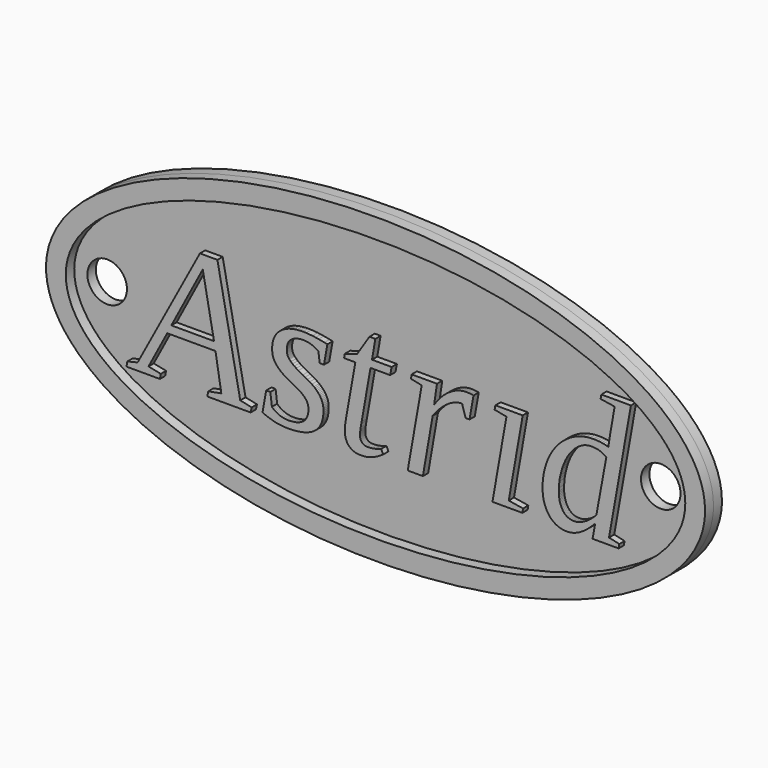
from build123d import *

# Parameters (mm, degrees)
F0_R     = 3
F1_DEPTH = 1.6
F2_DEPTH = 1.6
F3_DEPTH = 1


# Not quite as in the source:
# - a feature names something its author has since deleted; it is built from what else it names


with BuildPart() as f1:
    # F0 (on Front) → F1 (new body)
    with BuildSketch(Plane.XZ):
        with BuildLine():
            add(Edge.make_bspline(
                [(50, 0), (50, 39.8371685741), (-25, 19.918584287), (-100, 0), (-25, -19.918584287), (50, -39.8371685741), (50, 0)],
                knots=[0, 0, 0, 2.0943951024, 2.0943951024, 4.1887902048, 4.1887902048, 6.2831853072, 6.2831853072, 6.2831853072], degree=2, weights=[1, 0.5, 1, 0.5, 1, 0.5, 1]))
        make_face()
        with BuildLine():
            add(Edge.make_bspline(
                [(47, 0), (47, 34.6410161514), (-23.5, 17.3205080757), (-94, 0), (-23.5, -17.3205080757), (47, -34.6410161514), (47, 0)],
                knots=[0, 0, 0, 2.0943951024, 2.0943951024, 4.1887902048, 4.1887902048, 6.2831853072, 6.2831853072, 6.2831853072], degree=2, weights=[1, 0.5, 1, 0.5, 1, 0.5, 1]))
        make_face(mode=Mode.SUBTRACT)
        with BuildLine():
            add(Edge.make_bspline(
                [(47, 0), (47, 34.6410161514), (-23.5, 17.3205080757), (-94, 0), (-23.5, -17.3205080757), (47, -34.6410161514), (47, 0)],
                knots=[0, 0, 0, 2.0943951024, 2.0943951024, 4.1887902048, 4.1887902048, 6.2831853072, 6.2831853072, 6.2831853072], degree=2, weights=[1, 0.5, 1, 0.5, 1, 0.5, 1]))
        make_face()
        Polygon((-34.93235, -8.5991), (-33.05995, -8.9736), (-33.19865, -9.7087), (-38.27495, -9.7087), (-38.13625, -8.9736), (-36.58285, -8.5991), (-27.12375, 9.043), (-24.47465, 9.043), (-21.00725, -8.5991), (-19.27355, -8.9736), (-19.42615, -9.7087), (-26.01425, -9.7087), (-25.86165, -8.9736), (-23.87825, -8.5991), (-24.76595, -3.2316), (-32.08905, -3.2316), align=None, mode=Mode.SUBTRACT)
        Polygon((-8.39175, -5.6462), (-8.38525, -5.8807), (-8.39045, -6.1382), (-8.40605, -6.3874), (-8.43205, -6.628), (-8.46845, -6.8602), (-8.51525, -7.084), (-8.57245, -7.2993), (-8.64005, -7.5061), (-8.71805, -7.7045), (-8.80655, -7.8945), (-8.90535, -8.076), (-9.01455, -8.249), (-9.13415, -8.4136), (-9.26425, -8.5698), (-9.40465, -8.7175), (-9.55545, -8.8567), (-9.71665, -8.9875), (-9.88845, -9.1084), (-10.07105, -9.2215), (-10.26425, -9.3269), (-10.46825, -9.4244), (-10.68295, -9.5141), (-10.90845, -9.596), (-11.14455, -9.6701), (-11.39145, -9.7364), (-11.64905, -9.795), (-11.91745, -9.8457), (-12.19645, -9.8886), (-12.48625, -9.9237), (-13.09805, -9.9705), (-13.75275, -9.9861), (-14.36045, -9.9688), (-14.93515, -9.9167), (-15.47695, -9.8301), (-15.73545, -9.7737), (-15.98575, -9.7087), (-16.45825, -9.5631), (-16.67945, -9.4903), (-16.89075, -9.4174), (-17.09205, -9.3446), (-17.28345, -9.2718), (-17.46485, -9.199), (-17.63625, -9.1262), (-17.06755, -5.9916), (-16.44345, -5.9916), (-16.20765, -7.8918), (-16.11295, -7.9876), (-16.00915, -8.0808), (-15.89625, -8.1713), (-15.77425, -8.2593), (-15.64315, -8.3447), (-15.50295, -8.4275), (-15.35365, -8.5077), (-15.19515, -8.5853), (-15.02615, -8.6568), (-14.85195, -8.7188), (-14.67245, -8.7712), (-14.48785, -8.8141), (-14.29805, -8.8475), (-14.10295, -8.8713), (-13.90275, -8.8856), (-13.69725, -8.8904), (-13.38955, -8.8826), (-13.09045, -8.8592), (-12.80005, -8.8202), (-12.51835, -8.7656), (-12.38185, -8.732), (-12.24965, -8.6936), (-12.12175, -8.6505), (-11.99825, -8.6026), (-11.87905, -8.5499), (-11.76425, -8.4925), (-11.65365, -8.4303), (-11.54745, -8.3633), (-11.44625, -8.2877), (-11.35075, -8.2064), (-11.26075, -8.1195), (-11.17645, -8.027), (-11.09785, -7.9288), (-11.02475, -7.825), (-10.95735, -7.7156), (-10.89565, -7.6005), (-10.84035, -7.4757), (-10.79245, -7.3439), (-10.75195, -7.2052), (-10.71875, -7.0596), (-10.69295, -6.907), (-10.67455, -6.7475), (-10.66355, -6.5811), (-10.65985, -6.4077), (-10.66635, -6.2311), (-10.67445, -6.1456), (-10.68585, -6.0619), (-10.70045, -5.98), (-10.71835, -5.9), (-10.73945, -5.8218), (-10.76385, -5.7455), (-10.79145, -5.671), (-10.82235, -5.5983), (-10.85655, -5.5275), (-10.89385, -5.4585), (-10.93455, -5.3914), (-10.97845, -5.3261), (-11.02555, -5.2627), (-11.07595, -5.2011), (-11.17975, -5.0814), (-11.29005, -4.9653), (-11.40685, -4.8526), (-11.53015, -4.7434), (-11.65995, -4.6376), (-11.93905, -4.4365), (-12.08845, -4.3412), (-12.40045, -4.1496), (-13.06625, -3.782), (-13.41985, -3.6061), (-13.76745, -3.4266), (-14.10295, -3.2351), (-14.42635, -3.0313), (-14.73755, -2.8155), (-15.03045, -2.5762), (-15.29925, -2.3162), (-15.54365, -2.0353), (-15.76385, -1.7337), (-15.85815, -1.5726), (-15.93985, -1.4017), (-16.00895, -1.2207), (-16.06555, -1.0298), (-16.10955, -0.8289), (-16.14095, -0.618), (-16.15975, -0.3972), (-16.16605, -0.1664), (-16.16025, 0.0889), (-16.14265, 0.3346), (-16.11345, 0.5709), (-16.07245, 0.7975), (-16.01975, 1.0147), (-15.95545, 1.2223), (-15.87935, 1.4204), (-15.79155, 1.6089), (-15.69065, 1.7884), (-15.58185, 1.9591), (-15.46525, 2.1212), (-15.34085, 2.2747), (-15.20865, 2.4194), (-15.06865, 2.5555), (-14.92085, 2.6829), (-14.76525, 2.8017), (-14.59945, 2.9122), (-14.42805, 3.0149), (-14.25095, 3.1099), (-14.06825, 3.197), (-13.87995, 3.2763), (-13.68605, 3.3478), (-13.48645, 3.4115), (-13.28115, 3.4674), (-12.85295, 3.5585), (-12.41435, 3.6235), (-11.96535, 3.6625), (-11.50585, 3.6755), (-11.01095, 3.666), (-10.04695, 3.5897), (-9.57805, 3.5229), (-9.11775, 3.4501), (-8.22315, 3.2837), (-7.78885, 3.1901), (-8.30195, 0.2913), (-8.95385, 0.2913), (-9.14805, 1.7892), (-9.24855, 1.8737), (-9.35605, 1.9539), (-9.47055, 2.0298), (-9.59185, 2.1013), (-9.72015, 2.1685), (-9.85535, 2.2313), (-9.99755, 2.2898), (-10.14665, 2.344), (-10.29745, 2.396), (-10.45175, 2.4411), (-10.60955, 2.4792), (-10.77075, 2.5104), (-10.93545, 2.5347), (-11.10365, 2.552), (-11.27525, 2.5625), (-11.45045, 2.5659), (-11.72755, 2.5577), (-11.99045, 2.533), (-12.23905, 2.4918), (-12.35795, 2.465), (-12.47325, 2.4342), (-12.58505, 2.3992), (-12.69325, 2.36), (-12.79785, 2.3168), (-12.89895, 2.2695), (-12.99635, 2.218), (-13.09025, 2.1624), (-13.18055, 2.1027), (-13.26735, 2.0389), (-13.34965, 1.9725), (-13.42665, 1.9015), (-13.49825, 1.826), (-13.56465, 1.7459), (-13.62575, 1.6613), (-13.68145, 1.5721), (-13.73185, 1.4783), (-13.77705, 1.3801), (-13.81685, 1.2772), (-13.85135, 1.1699), (-13.88055, 1.0579), (-13.90445, 0.9414), (-13.92305, 0.8204), (-13.93635, 0.6948), (-13.94425, 0.5647), (-13.94695, 0.43), (-13.94065, 0.2636), (-13.93275, 0.1829), (-13.92175, 0.1041), (-13.90765, 0.0269), (-13.89035, -0.0485), (-13.86995, -0.1222), (-13.84635, -0.1941), (-13.81965, -0.2644), (-13.78985, -0.3328), (-13.75685, -0.3996), (-13.72065, -0.4646), (-13.68145, -0.5279), (-13.63895, -0.5894), (-13.59345, -0.6492), (-13.54475, -0.7073), (-13.32365, -0.9318), (-13.07665, -1.1477), (-12.80355, -1.3549), (-12.50445, -1.5534), (-12.18725, -1.7406), (-11.52145, -2.1151), (-11.17305, -2.3023), (-10.81845, -2.4896), (-10.47605, -2.6907), (-10.14575, -2.9056), (-9.82765, -3.1345), (-9.67505, -3.2554), (-9.52945, -3.3824), (-9.39075, -3.5155), (-9.25905, -3.6546), (-9.13415, -3.7998), (-9.01625, -3.9511), (-8.90535, -4.1084), (-8.80135, -4.2718), (-8.70375, -4.4395), (-8.61925, -4.6168), (-8.54775, -4.8036), (-8.48925, -5), (-8.44375, -5.2058), (-8.41125, -5.4213), align=None, mode=Mode.SUBTRACT)
        Polygon((-2.83555, -7.2163), (-2.83665, -7.2954), (-2.83545, -7.3722), (-2.83195, -7.4467), (-2.82595, -7.5187), (-2.81755, -7.5884), (-2.80685, -7.6557), (-2.79375, -7.7206), (-2.77825, -7.7831), (-2.76035, -7.8432), (-2.74015, -7.901), (-2.71745, -7.9564), (-2.69245, -8.0093), (-2.66505, -8.0599), (-2.63525, -8.1082), (-2.60305, -8.154), (-2.56845, -8.1975), (-2.53155, -8.2385), (-2.49105, -8.2755), (-2.44915, -8.31), (-2.40605, -8.3422), (-2.36165, -8.372), (-2.31595, -8.3994), (-2.26885, -8.4245), (-2.22055, -8.4471), (-2.17095, -8.4674), (-2.12005, -8.4852), (-2.06775, -8.5007), (-2.01425, -8.5139), (-1.95945, -8.5246), (-1.90325, -8.5329), (-1.84585, -8.5389), (-1.78715, -8.5425), (-1.72715, -8.5437), (-1.43495, -8.5367), (-1.15495, -8.5159), (-0.88715, -8.4812), (-0.63145, -8.4327), (-0.38085, -8.372), (0.12535, -8.2194), (0.38105, -8.1276), (0.67235, -8.7794), (0.30995, -9.0204), (-0.06965, -9.2441), (-0.46665, -9.4504), (-0.88105, -9.6394), (-1.09275, -9.7206), (-1.31185, -9.7911), (-1.53835, -9.8506), (-1.77215, -9.8994), (-2.01335, -9.9373), (-2.26195, -9.9644), (-2.51785, -9.9807), (-2.78115, -9.9861), (-2.92465, -9.9831), (-3.06375, -9.974), (-3.19855, -9.9588), (-3.32905, -9.9375), (-3.45515, -9.9102), (-3.57695, -9.8769), (-3.69445, -9.8374), (-3.80755, -9.7919), (-3.91635, -9.7445), (-4.02075, -9.6922), (-4.12095, -9.6352), (-4.21675, -9.5735), (-4.30815, -9.5069), (-4.39525, -9.4356), (-4.47805, -9.3596), (-4.55655, -9.2787), (-4.62715, -9.1936), (-4.69345, -9.1045), (-4.75545, -9.0115), (-4.81305, -8.9147), (-4.86645, -8.8139), (-4.91535, -8.7092), (-4.96005, -8.6006), (-5.00035, -8.4882), (-5.06105, -8.2472), (-5.10435, -7.9958), (-5.13035, -7.734), (-5.13905, -7.4618), (-5.13465, -7.2538), (-5.12165, -7.0319), (-5.10005, -6.7961), (-5.06965, -6.5464), (-5.03415, -6.2924), (-4.95785, -5.8001), (-4.91715, -5.5617), (-3.54405, 2.1637), (-5.24995, 2.1637), (-5.13905, 2.7878), (-3.29435, 3.3287), (-1.39425, 6.283), (-0.50655, 6.283), (-1.01975, 3.3287), (1.96225, 3.3287), (1.74035, 2.1637), (-1.24165, 2.1637), (-2.58705, -5.4507), (-2.63985, -5.7299), (-2.73005, -6.2569), (-2.76735, -6.5048), (-2.78355, -6.6234), (-2.79765, -6.7363), (-2.80955, -6.8435), (-2.81935, -6.9452), (-2.82695, -7.0412), (-2.83235, -7.1315), align=None, mode=Mode.SUBTRACT)
        Polygon((13.14785, 3.6722), (13.29435, 3.6755), (13.43655, 3.6729), (13.58565, 3.6651), (13.74165, 3.6521), (13.90465, 3.6339), (13.98505, 3.6267), (14.05985, 3.6191), (14.12895, 3.6111), (14.16145, 3.607), (14.19245, 3.6027), (14.22205, 3.5983), (14.25035, 3.5938), (14.27715, 3.5892), (14.30255, 3.5845), (14.32655, 3.5796), (14.34915, 3.5747), (14.37035, 3.5697), (14.39005, 3.5645), (13.77985, 0.1526), (13.18345, 0.1526), (12.65635, 1.914), (12.50385, 1.9101), (12.35125, 1.8984), (12.19865, 1.8789), (12.04615, 1.8516), (11.89355, 1.8165), (11.74095, 1.7736), (11.58845, 1.7229), (11.43585, 1.6644), (11.13335, 1.5283), (10.83605, 1.3697), (10.54385, 1.1885), (10.25695, 0.9848), (9.97525, 0.7681), (9.69865, 0.534), (9.42735, 0.2826), (9.16125, 0.0139), (8.90295, -0.2678), (8.41745, -0.8573), (8.19035, -1.165), (6.70635, -9.7087), (4.40395, -9.7087), (6.52605, 2.3579), (4.88945, 2.7046), (5.00035, 3.3287), (8.84225, 3.3287), (8.41225, 0.3884), (8.69315, 0.7915), (8.98095, 1.1686), (9.27565, 1.5196), (9.57735, 1.8447), (9.88945, 2.1429), (10.20145, 2.4134), (10.51355, 2.6561), (10.82565, 2.871), (11.13765, 3.0592), (11.44975, 3.2213), (11.76185, 3.3574), (12.07385, 3.4674), (12.38945, 3.5585), (12.69805, 3.6235), (12.84975, 3.6462), (12.99965, 3.6625), align=None, mode=Mode.SUBTRACT)
        Polygon((21.85265, 3.3287), (19.73055, -8.7378), (21.90815, -9.0846), (21.79715, -9.7087), (17.26185, -9.7087), (19.38385, 2.3579), (17.59465, 2.7046), (17.70565, 3.3287), align=None, mode=Mode.SUBTRACT)
        with Locations((-42, 0)):
            Circle(F0_R, mode=Mode.SUBTRACT)
        Polygon((22.71065, 7.6626), (22.71255, 7.5867), (22.71065, 7.5109), (22.70475, 7.4359), (22.69505, 7.3618), (22.68135, 7.2885), (22.66385, 7.2161), (22.64235, 7.1446), (22.61695, 7.074), (22.58775, 7.0042), (22.55845, 6.9392), (22.52615, 6.8759), (22.49085, 6.8144), (22.45255, 6.7545), (22.41115, 6.6965), (22.36665, 6.6401), (22.31925, 6.5855), (22.26875, 6.5326), (22.21565, 6.4819), (22.16035, 6.4338), (22.10295, 6.3883), (22.04335, 6.3454), (21.98155, 6.3051), (21.91765, 6.2674), (21.85155, 6.2323), (21.78325, 6.1998), (21.71355, 6.1738), (21.64285, 6.1512), (21.57135, 6.1321), (21.49895, 6.1165), (21.42575, 6.1044), (21.35165, 6.0957), (21.27665, 6.0905), (21.20075, 6.0888), (21.12495, 6.0905), (21.04995, 6.0957), (20.97585, 6.1044), (20.90255, 6.1165), (20.83015, 6.1321), (20.75865, 6.1512), (20.68805, 6.1738), (20.61825, 6.1998), (20.48995, 6.2674), (20.36855, 6.3454), (20.25415, 6.4338), (20.14665, 6.5326), (20.04785, 6.6401), (19.95945, 6.7545), (19.88145, 6.8759), (19.81385, 7.0042), (19.78785, 7.074), (19.76525, 7.1446), (19.74615, 7.2161), (19.73055, 7.2885), (19.71845, 7.3618), (19.70975, 7.4359), (19.70455, 7.5109), (19.70285, 7.5867), (19.70455, 7.6626), (19.70975, 7.7376), (19.71845, 7.8117), (19.73055, 7.8849), (19.74615, 7.9573), (19.76525, 8.0288), (19.78785, 8.0995), (19.81385, 8.1692), (19.84635, 8.2375), (19.88145, 8.3036), (19.91915, 8.3675), (19.95945, 8.4293), (20.00235, 8.4889), (20.04785, 8.5463), (20.09595, 8.6016), (20.14665, 8.6547), (20.19955, 8.7052), (20.25415, 8.7526), (20.31055, 8.7971), (20.36855, 8.8385), (20.42845, 8.8768), (20.48995, 8.9121), (20.55325, 8.9444), (20.61825, 8.9737), (20.68805, 9.0029), (20.75865, 9.0283), (20.83015, 9.0497), (20.90255, 9.0673), (20.97585, 9.081), (21.04995, 9.0907), (21.12495, 9.0966), (21.20075, 9.0985), (21.27665, 9.0966), (21.35165, 9.0907), (21.42575, 9.081), (21.49895, 9.0673), (21.57135, 9.0497), (21.64285, 9.0283), (21.71355, 9.0029), (21.78325, 8.9737), (21.85155, 8.9444), (21.91765, 8.9121), (21.98155, 8.8768), (22.04335, 8.8385), (22.10295, 8.7971), (22.16035, 8.7526), (22.21565, 8.7052), (22.26875, 8.6547), (22.31925, 8.6016), (22.36665, 8.5463), (22.41115, 8.4889), (22.45255, 8.4293), (22.49085, 8.3675), (22.52615, 8.3036), (22.55845, 8.2375), (22.58775, 8.1692), (22.61695, 8.0995), (22.64235, 8.0288), (22.66385, 7.9573), (22.68135, 7.8849), (22.69505, 7.8117), (22.70475, 7.7376), align=None, mode=Mode.SUBTRACT)
        Polygon((34.62115, 3.4146), (34.86305, 3.3426), (34.86485, 3.364), (34.86695, 3.3864), (34.86925, 3.4099), (34.87175, 3.4345), (34.87735, 3.4869), (34.88385, 3.5437), (34.89125, 3.6048), (34.89945, 3.6703), (34.90855, 3.7401), (34.91855, 3.8142), (34.94015, 3.9746), (34.98875, 4.3005), (35.01565, 4.4661), (35.04245, 4.6377), (35.09105, 4.9706), (35.11275, 5.1318), (35.12635, 5.2098), (35.13955, 5.2844), (35.15235, 5.3554), (35.16475, 5.4231), (35.17665, 5.4872), (35.18815, 5.5479), (35.19915, 5.6051), (35.20975, 5.6588), (35.80615, 9.043), (33.67025, 9.3759), (33.78125, 10), (38.27495, 10), (34.94625, -8.7378), (36.51355, -9.0846), (36.40255, -9.7087), (32.44975, -9.7087), (32.85195, -7.545), (32.56225, -7.8409), (32.27545, -8.118), (31.99185, -8.3766), (31.71115, -8.6165), (31.43355, -8.8377), (31.15895, -9.0404), (30.88745, -9.2243), (30.61895, -9.3897), (30.35325, -9.5327), (30.09015, -9.6567), (29.82965, -9.7616), (29.57175, -9.8474), (29.31645, -9.9141), (29.06385, -9.9618), (28.81375, -9.9904), (28.56625, -10), (28.36055, -9.995), (28.15965, -9.98), (27.96355, -9.9551), (27.77225, -9.9202), (27.58565, -9.8754), (27.40375, -9.8205), (27.22675, -9.7557), (27.05445, -9.681), (26.88755, -9.5969), (26.72675, -9.5041), (26.57205, -9.4027), (26.42335, -9.2926), (26.28075, -9.1739), (26.14425, -9.0464), (26.01375, -8.9103), (25.88945, -8.7656), (25.77125, -8.6089), (25.65965, -8.444), (25.55455, -8.2708), (25.45595, -8.0894), (25.36385, -7.8998), (25.27825, -7.7019), (25.19915, -7.4958), (25.12655, -7.2815), (25.06485, -7.0596), (25.01125, -6.8308), (24.96595, -6.595), (24.90015, -6.1026), (24.86715, -5.5825), (24.86305, -5.312), (24.87955, -4.72), (24.92895, -4.1366), (25.01125, -3.5619), (25.12655, -2.9958), (25.27225, -2.4358), (25.44555, -1.8932), (25.64665, -1.3679), (25.87555, -0.8599), (26.13035, -0.3718), (26.40955, 0.0937), (26.71295, 0.5366), (27.04055, 0.957), (27.39775, 1.3584), (27.77565, 1.7303), (28.17445, 2.0727), (28.59395, 2.3856), (29.03265, 2.6734), (29.48855, 2.9265), (29.96185, 3.145), (30.45255, 3.3287), (30.96485, 3.4744), (31.48925, 3.5784), (32.02585, 3.6408), (32.57455, 3.6616), (32.91265, 3.6564), (33.23335, 3.6408), (33.53675, 3.6148), (33.82285, 3.5784), (34.10105, 3.5325), (34.36725, 3.4778), align=None, mode=Mode.SUBTRACT)
        with Locations((42, 0)):
            Circle(F0_R, mode=Mode.SUBTRACT)
        Polygon((34.86485, 3.364), (34.86305, 3.3426), (34.62115, 3.4146), (34.36725, 3.4778), (34.10105, 3.5325), (33.82285, 3.5784), (33.53675, 3.6148), (33.23335, 3.6408), (32.91265, 3.6564), (32.57455, 3.6616), (32.02585, 3.6408), (31.48925, 3.5784), (30.96485, 3.4744), (30.45255, 3.3287), (29.96185, 3.145), (29.48855, 2.9265), (29.03265, 2.6734), (28.59395, 2.3856), (28.17445, 2.0727), (27.77565, 1.7303), (27.39775, 1.3584), (27.04055, 0.957), (26.71295, 0.5366), (26.40955, 0.0937), (26.13035, -0.3718), (25.87555, -0.8599), (25.64665, -1.3679), (25.44555, -1.8932), (25.27225, -2.4358), (25.12655, -2.9958), (25.01125, -3.5619), (24.92895, -4.1366), (24.87955, -4.72), (24.86305, -5.312), (24.86715, -5.5825), (24.90015, -6.1026), (24.96595, -6.595), (25.01125, -6.8308), (25.06485, -7.0596), (25.12655, -7.2815), (25.19915, -7.4958), (25.27825, -7.7019), (25.36385, -7.8998), (25.45595, -8.0894), (25.55455, -8.2708), (25.65965, -8.444), (25.77125, -8.6089), (25.88945, -8.7656), (26.01375, -8.9103), (26.14425, -9.0464), (26.28075, -9.1739), (26.42335, -9.2926), (26.57205, -9.4027), (26.72675, -9.5041), (26.88755, -9.5969), (27.05445, -9.681), (27.22675, -9.7557), (27.40375, -9.8205), (27.58565, -9.8754), (27.77225, -9.9202), (27.96355, -9.9551), (28.15965, -9.98), (28.36055, -9.995), (28.56625, -10), (28.81375, -9.9904), (29.06385, -9.9618), (29.31645, -9.9141), (29.57175, -9.8474), (29.82965, -9.7616), (30.09015, -9.6567), (30.35325, -9.5327), (30.61895, -9.3897), (30.88745, -9.2243), (31.15895, -9.0404), (31.43355, -8.8377), (31.71115, -8.6165), (31.99185, -8.3766), (32.27545, -8.118), (32.56225, -7.8409), (32.85195, -7.545), (32.44975, -9.7087), (36.40255, -9.7087), (36.51355, -9.0846), (34.94625, -8.7378), (38.27495, 10), (33.78125, 10), (33.67025, 9.3759), (35.80615, 9.043), (35.20975, 5.6588), (35.19915, 5.6051), (35.18815, 5.5479), (35.17665, 5.4872), (35.16475, 5.4231), (35.15235, 5.3554), (35.13955, 5.2844), (35.12635, 5.2098), (35.11275, 5.1318), (35.09105, 4.9706), (35.04245, 4.6377), (35.01565, 4.4661), (34.98875, 4.3005), (34.94015, 3.9746), (34.91855, 3.8142), (34.90855, 3.7401), (34.89945, 3.6703), (34.89125, 3.6048), (34.88385, 3.5437), (34.87735, 3.4869), (34.87175, 3.4345), (34.86925, 3.4099), (34.86695, 3.3864), align=None)
        Polygon((34.29955, 2.051), (34.54405, 1.9002), (33.03225, -6.3384), (32.81965, -6.5609), (32.38795, -6.9684), (32.16885, -7.1532), (31.94765, -7.3255), (31.72415, -7.4852), (31.49855, -7.6324), (31.27085, -7.767), (31.04735, -7.884), (30.82785, -7.9854), (30.61225, -8.0712), (30.40045, -8.1414), (30.19265, -8.196), (29.98875, -8.2351), (29.78875, -8.2585), (29.59255, -8.2663), (29.48535, -8.2634), (29.37845, -8.255), (29.27205, -8.2409), (29.16615, -8.2212), (29.06055, -8.1958), (28.95545, -8.1648), (28.85075, -8.1282), (28.74655, -8.086), (28.64725, -8.0376), (28.55065, -7.9828), (28.45655, -7.9215), (28.36515, -7.8536), (28.27625, -7.7793), (28.19005, -7.6985), (28.10635, -7.6111), (28.02535, -7.5173), (27.95075, -7.4135), (27.87965, -7.3032), (27.81205, -7.1864), (27.74795, -7.0631), (27.68725, -6.9333), (27.63005, -6.7969), (27.57625, -6.6541), (27.52605, -6.5048), (27.48055, -6.3449), (27.44105, -6.1771), (27.40765, -6.0016), (27.38035, -5.8183), (27.35915, -5.6271), (27.34395, -5.4282), (27.33485, -5.2214), (27.33185, -5.0069), (27.34135, -4.5622), (27.41765, -3.6676), (27.48445, -3.2177), (27.57625, -2.7704), (27.81205, -1.8966), (27.95595, -1.4701), (28.11635, -1.0541), (28.29235, -0.6518), (28.48385, -0.2635), (28.69105, 0.111), (28.91995, 0.4664), (29.16265, 0.7975), (29.41925, 1.1044), (29.68965, 1.387), (29.82985, 1.522), (30.11945, 1.7699), (30.42105, 1.9884), (30.73485, 2.1774), (30.89635, 2.2608), (31.06085, 2.3356), (31.22835, 2.4004), (31.39885, 2.4552), (31.57245, 2.5), (31.74915, 2.5349), (31.92875, 2.5599), (32.11145, 2.5748), (32.29715, 2.5798), (32.47745, 2.577), (32.65085, 2.5685), (32.81725, 2.5544), (32.97675, 2.5347), (33.12935, 2.5094), (33.27495, 2.4784), (33.41365, 2.4417), (33.54545, 2.3995), (33.80025, 2.3007), (34.05165, 2.1845), align=None, mode=Mode.SUBTRACT)
        Polygon((-33.19865, -9.7087), (-33.05995, -8.9736), (-34.93235, -8.5991), (-32.08905, -3.2316), (-24.76595, -3.2316), (-23.87825, -8.5991), (-25.86165, -8.9736), (-26.01425, -9.7087), (-19.42615, -9.7087), (-19.27355, -8.9736), (-21.00725, -8.5991), (-24.47465, 9.043), (-27.12375, 9.043), (-36.58285, -8.5991), (-38.13625, -8.9736), (-38.27495, -9.7087), align=None)
        Polygon((-31.46495, -1.9833), (-26.69385, 7.0458), (-24.98785, -1.9833), align=None, mode=Mode.SUBTRACT)
        Polygon((33.03225, -6.3384), (34.54405, 1.9002), (34.29955, 2.051), (34.05165, 2.1845), (33.80025, 2.3007), (33.54545, 2.3995), (33.41365, 2.4417), (33.27495, 2.4784), (33.12935, 2.5094), (32.97675, 2.5347), (32.81725, 2.5544), (32.65085, 2.5685), (32.47745, 2.577), (32.29715, 2.5798), (32.11145, 2.5748), (31.92875, 2.5599), (31.74915, 2.5349), (31.57245, 2.5), (31.39885, 2.4552), (31.22835, 2.4004), (31.06085, 2.3356), (30.89635, 2.2608), (30.73485, 2.1774), (30.42105, 1.9884), (30.11945, 1.7699), (29.82985, 1.522), (29.68965, 1.387), (29.41925, 1.1044), (29.16265, 0.7975), (28.91995, 0.4664), (28.69105, 0.111), (28.48385, -0.2635), (28.29235, -0.6518), (28.11635, -1.0541), (27.95595, -1.4701), (27.81205, -1.8966), (27.57625, -2.7704), (27.48445, -3.2177), (27.41765, -3.6676), (27.34135, -4.5622), (27.33185, -5.0069), (27.33485, -5.2214), (27.34395, -5.4282), (27.35915, -5.6271), (27.38035, -5.8183), (27.40765, -6.0016), (27.44105, -6.1771), (27.48055, -6.3449), (27.52605, -6.5048), (27.57625, -6.6541), (27.63005, -6.7969), (27.68725, -6.9333), (27.74795, -7.0631), (27.81205, -7.1864), (27.87965, -7.3032), (27.95075, -7.4135), (28.02535, -7.5173), (28.10635, -7.6111), (28.19005, -7.6985), (28.27625, -7.7793), (28.36515, -7.8536), (28.45655, -7.9215), (28.55065, -7.9828), (28.64725, -8.0376), (28.74655, -8.086), (28.85075, -8.1282), (28.95545, -8.1648), (29.06055, -8.1958), (29.16615, -8.2212), (29.27205, -8.2409), (29.37845, -8.255), (29.48535, -8.2634), (29.59255, -8.2663), (29.78875, -8.2585), (29.98875, -8.2351), (30.19265, -8.196), (30.40045, -8.1414), (30.61225, -8.0712), (30.82785, -7.9854), (31.04735, -7.884), (31.27085, -7.767), (31.49855, -7.6324), (31.72415, -7.4852), (31.94765, -7.3255), (32.16885, -7.1532), (32.38795, -6.9684), (32.81965, -6.5609), align=None)
        Polygon((-8.39045, -6.1382), (-8.38525, -5.8807), (-8.39175, -5.6462), (-8.41125, -5.4213), (-8.44375, -5.2058), (-8.48925, -5), (-8.54775, -4.8036), (-8.61925, -4.6168), (-8.70375, -4.4395), (-8.80135, -4.2718), (-8.90535, -4.1084), (-9.01625, -3.9511), (-9.13415, -3.7998), (-9.25905, -3.6546), (-9.39075, -3.5155), (-9.52945, -3.3824), (-9.67505, -3.2554), (-9.82765, -3.1345), (-10.14575, -2.9056), (-10.47605, -2.6907), (-10.81845, -2.4896), (-11.17305, -2.3023), (-11.52145, -2.1151), (-12.18725, -1.7406), (-12.50445, -1.5534), (-12.80355, -1.3549), (-13.07665, -1.1477), (-13.32365, -0.9318), (-13.54475, -0.7073), (-13.59345, -0.6492), (-13.63895, -0.5894), (-13.68145, -0.5279), (-13.72065, -0.4646), (-13.75685, -0.3996), (-13.78985, -0.3328), (-13.81965, -0.2644), (-13.84635, -0.1941), (-13.86995, -0.1222), (-13.89035, -0.0485), (-13.90765, 0.0269), (-13.92175, 0.1041), (-13.93275, 0.1829), (-13.94065, 0.2636), (-13.94695, 0.43), (-13.94425, 0.5647), (-13.93635, 0.6948), (-13.92305, 0.8204), (-13.90445, 0.9414), (-13.88055, 1.0579), (-13.85135, 1.1699), (-13.81685, 1.2772), (-13.77705, 1.3801), (-13.73185, 1.4783), (-13.68145, 1.5721), (-13.62575, 1.6613), (-13.56465, 1.7459), (-13.49825, 1.826), (-13.42665, 1.9015), (-13.34965, 1.9725), (-13.26735, 2.0389), (-13.18055, 2.1027), (-13.09025, 2.1624), (-12.99635, 2.218), (-12.89895, 2.2695), (-12.79785, 2.3168), (-12.69325, 2.36), (-12.58505, 2.3992), (-12.47325, 2.4342), (-12.35795, 2.465), (-12.23905, 2.4918), (-11.99045, 2.533), (-11.72755, 2.5577), (-11.45045, 2.5659), (-11.27525, 2.5625), (-11.10365, 2.552), (-10.93545, 2.5347), (-10.77075, 2.5104), (-10.60955, 2.4792), (-10.45175, 2.4411), (-10.29745, 2.396), (-10.14665, 2.344), (-9.99755, 2.2898), (-9.85535, 2.2313), (-9.72015, 2.1685), (-9.59185, 2.1013), (-9.47055, 2.0298), (-9.35605, 1.9539), (-9.24855, 1.8737), (-9.14805, 1.7892), (-8.95385, 0.2913), (-8.30195, 0.2913), (-7.78885, 3.1901), (-8.22315, 3.2837), (-9.11775, 3.4501), (-9.57805, 3.5229), (-10.04695, 3.5897), (-11.01095, 3.666), (-11.50585, 3.6755), (-11.96535, 3.6625), (-12.41435, 3.6235), (-12.85295, 3.5585), (-13.28115, 3.4674), (-13.48645, 3.4115), (-13.68605, 3.3478), (-13.87995, 3.2763), (-14.06825, 3.197), (-14.25095, 3.1099), (-14.42805, 3.0149), (-14.59945, 2.9122), (-14.76525, 2.8017), (-14.92085, 2.6829), (-15.06865, 2.5555), (-15.20865, 2.4194), (-15.34085, 2.2747), (-15.46525, 2.1212), (-15.58185, 1.9591), (-15.69065, 1.7884), (-15.79155, 1.6089), (-15.87935, 1.4204), (-15.95545, 1.2223), (-16.01975, 1.0147), (-16.07245, 0.7975), (-16.11345, 0.5709), (-16.14265, 0.3346), (-16.16025, 0.0889), (-16.16605, -0.1664), (-16.15975, -0.3972), (-16.14095, -0.618), (-16.10955, -0.8289), (-16.06555, -1.0298), (-16.00895, -1.2207), (-15.93985, -1.4017), (-15.85815, -1.5726), (-15.76385, -1.7337), (-15.54365, -2.0353), (-15.29925, -2.3162), (-15.03045, -2.5762), (-14.73755, -2.8155), (-14.42635, -3.0313), (-14.10295, -3.2351), (-13.76745, -3.4266), (-13.41985, -3.6061), (-13.06625, -3.782), (-12.40045, -4.1496), (-12.08845, -4.3412), (-11.93905, -4.4365), (-11.65995, -4.6376), (-11.53015, -4.7434), (-11.40685, -4.8526), (-11.29005, -4.9653), (-11.17975, -5.0814), (-11.07595, -5.2011), (-11.02555, -5.2627), (-10.97845, -5.3261), (-10.93455, -5.3914), (-10.89385, -5.4585), (-10.85655, -5.5275), (-10.82235, -5.5983), (-10.79145, -5.671), (-10.76385, -5.7455), (-10.73945, -5.8218), (-10.71835, -5.9), (-10.70045, -5.98), (-10.68585, -6.0619), (-10.67445, -6.1456), (-10.66635, -6.2311), (-10.65985, -6.4077), (-10.66355, -6.5811), (-10.67455, -6.7475), (-10.69295, -6.907), (-10.71875, -7.0596), (-10.75195, -7.2052), (-10.79245, -7.3439), (-10.84035, -7.4757), (-10.89565, -7.6005), (-10.95735, -7.7156), (-11.02475, -7.825), (-11.09785, -7.9288), (-11.17645, -8.027), (-11.26075, -8.1195), (-11.35075, -8.2064), (-11.44625, -8.2877), (-11.54745, -8.3633), (-11.65365, -8.4303), (-11.76425, -8.4925), (-11.87905, -8.5499), (-11.99825, -8.6026), (-12.12175, -8.6505), (-12.24965, -8.6936), (-12.38185, -8.732), (-12.51835, -8.7656), (-12.80005, -8.8202), (-13.09045, -8.8592), (-13.38955, -8.8826), (-13.69725, -8.8904), (-13.90275, -8.8856), (-14.10295, -8.8713), (-14.29805, -8.8475), (-14.48785, -8.8141), (-14.67245, -8.7712), (-14.85195, -8.7188), (-15.02615, -8.6568), (-15.19515, -8.5853), (-15.35365, -8.5077), (-15.50295, -8.4275), (-15.64315, -8.3447), (-15.77425, -8.2593), (-15.89625, -8.1713), (-16.00915, -8.0808), (-16.11295, -7.9876), (-16.20765, -7.8918), (-16.44345, -5.9916), (-17.06755, -5.9916), (-17.63625, -9.1262), (-17.46485, -9.199), (-17.28345, -9.2718), (-17.09205, -9.3446), (-16.89075, -9.4174), (-16.67945, -9.4903), (-16.45825, -9.5631), (-15.98575, -9.7087), (-15.73545, -9.7737), (-15.47695, -9.8301), (-14.93515, -9.9167), (-14.36045, -9.9688), (-13.75275, -9.9861), (-13.09805, -9.9705), (-12.48625, -9.9237), (-12.19645, -9.8886), (-11.91745, -9.8457), (-11.64905, -9.795), (-11.39145, -9.7364), (-11.14455, -9.6701), (-10.90845, -9.596), (-10.68295, -9.5141), (-10.46825, -9.4244), (-10.26425, -9.3269), (-10.07105, -9.2215), (-9.88845, -9.1084), (-9.71665, -8.9875), (-9.55545, -8.8567), (-9.40465, -8.7175), (-9.26425, -8.5698), (-9.13415, -8.4136), (-9.01455, -8.249), (-8.90535, -8.076), (-8.80655, -7.8945), (-8.71805, -7.7045), (-8.64005, -7.5061), (-8.57245, -7.2993), (-8.51525, -7.084), (-8.46845, -6.8602), (-8.43205, -6.628), (-8.40605, -6.3874), align=None)
        Polygon((-2.83545, -7.3722), (-2.83665, -7.2954), (-2.83555, -7.2163), (-2.83235, -7.1315), (-2.82695, -7.0412), (-2.81935, -6.9452), (-2.80955, -6.8435), (-2.79765, -6.7363), (-2.78355, -6.6234), (-2.76735, -6.5048), (-2.73005, -6.2569), (-2.63985, -5.7299), (-2.58705, -5.4507), (-1.24165, 2.1637), (1.74035, 2.1637), (1.96225, 3.3287), (-1.01975, 3.3287), (-0.50655, 6.283), (-1.39425, 6.283), (-3.29435, 3.3287), (-5.13905, 2.7878), (-5.24995, 2.1637), (-3.54405, 2.1637), (-4.91715, -5.5617), (-4.95785, -5.8001), (-5.03415, -6.2924), (-5.06965, -6.5464), (-5.10005, -6.7961), (-5.12165, -7.0319), (-5.13465, -7.2538), (-5.13905, -7.4618), (-5.13035, -7.734), (-5.10435, -7.9958), (-5.06105, -8.2472), (-5.00035, -8.4882), (-4.96005, -8.6006), (-4.91535, -8.7092), (-4.86645, -8.8139), (-4.81305, -8.9147), (-4.75545, -9.0115), (-4.69345, -9.1045), (-4.62715, -9.1936), (-4.55655, -9.2787), (-4.47805, -9.3596), (-4.39525, -9.4356), (-4.30815, -9.5069), (-4.21675, -9.5735), (-4.12095, -9.6352), (-4.02075, -9.6922), (-3.91635, -9.7445), (-3.80755, -9.7919), (-3.69445, -9.8374), (-3.57695, -9.8769), (-3.45515, -9.9102), (-3.32905, -9.9375), (-3.19855, -9.9588), (-3.06375, -9.974), (-2.92465, -9.9831), (-2.78115, -9.9861), (-2.51785, -9.9807), (-2.26195, -9.9644), (-2.01335, -9.9373), (-1.77215, -9.8994), (-1.53835, -9.8506), (-1.31185, -9.7911), (-1.09275, -9.7206), (-0.88105, -9.6394), (-0.46665, -9.4504), (-0.06965, -9.2441), (0.30995, -9.0204), (0.67235, -8.7794), (0.38105, -8.1276), (0.12535, -8.2194), (-0.38085, -8.372), (-0.63145, -8.4327), (-0.88715, -8.4812), (-1.15495, -8.5159), (-1.43495, -8.5367), (-1.72715, -8.5437), (-1.78715, -8.5425), (-1.84585, -8.5389), (-1.90325, -8.5329), (-1.95945, -8.5246), (-2.01425, -8.5139), (-2.06775, -8.5007), (-2.12005, -8.4852), (-2.17095, -8.4674), (-2.22055, -8.4471), (-2.26885, -8.4245), (-2.31595, -8.3994), (-2.36165, -8.372), (-2.40605, -8.3422), (-2.44915, -8.31), (-2.49105, -8.2755), (-2.53155, -8.2385), (-2.56845, -8.1975), (-2.60305, -8.154), (-2.63525, -8.1082), (-2.66505, -8.0599), (-2.69245, -8.0093), (-2.71745, -7.9564), (-2.74015, -7.901), (-2.76035, -7.8432), (-2.77825, -7.7831), (-2.79375, -7.7206), (-2.80685, -7.6557), (-2.81755, -7.5884), (-2.82595, -7.5187), (-2.83195, -7.4467), align=None)
        Polygon((13.43655, 3.6729), (13.29435, 3.6755), (13.14785, 3.6722), (12.99965, 3.6625), (12.84975, 3.6462), (12.69805, 3.6235), (12.38945, 3.5585), (12.07385, 3.4674), (11.76185, 3.3574), (11.44975, 3.2213), (11.13765, 3.0592), (10.82565, 2.871), (10.51355, 2.6561), (10.20145, 2.4134), (9.88945, 2.1429), (9.57735, 1.8447), (9.27565, 1.5196), (8.98095, 1.1686), (8.69315, 0.7915), (8.41225, 0.3884), (8.84225, 3.3287), (5.00035, 3.3287), (4.88945, 2.7046), (6.52605, 2.3579), (4.40395, -9.7087), (6.70635, -9.7087), (8.19035, -1.165), (8.41745, -0.8573), (8.90295, -0.2678), (9.16125, 0.0139), (9.42735, 0.2826), (9.69865, 0.534), (9.97525, 0.7681), (10.25695, 0.9848), (10.54385, 1.1885), (10.83605, 1.3697), (11.13335, 1.5283), (11.43585, 1.6644), (11.58845, 1.7229), (11.74095, 1.7736), (11.89355, 1.8165), (12.04615, 1.8516), (12.19865, 1.8789), (12.35125, 1.8984), (12.50385, 1.9101), (12.65635, 1.914), (13.18345, 0.1526), (13.77985, 0.1526), (14.39005, 3.5645), (14.37035, 3.5697), (14.34915, 3.5747), (14.32655, 3.5796), (14.30255, 3.5845), (14.27715, 3.5892), (14.25035, 3.5938), (14.22205, 3.5983), (14.19245, 3.6027), (14.16145, 3.607), (14.12895, 3.6111), (14.05985, 3.6191), (13.98505, 3.6267), (13.90465, 3.6339), (13.74165, 3.6521), (13.58565, 3.6651), align=None)
        Polygon((21.90815, -9.0846), (19.73055, -8.7378), (21.85265, 3.3287), (17.70565, 3.3287), (17.59465, 2.7046), (19.38385, 2.3579), (17.26185, -9.7087), (21.79715, -9.7087), align=None)
        Polygon((-24.98785, -1.9833), (-26.69385, 7.0458), (-31.46495, -1.9833), align=None)
        Polygon((22.71065, 7.5109), (22.71255, 7.5867), (22.71065, 7.6626), (22.70475, 7.7376), (22.69505, 7.8117), (22.68135, 7.8849), (22.66385, 7.9573), (22.64235, 8.0288), (22.61695, 8.0995), (22.58775, 8.1692), (22.55845, 8.2375), (22.52615, 8.3036), (22.49085, 8.3675), (22.45255, 8.4293), (22.41115, 8.4889), (22.36665, 8.5463), (22.31925, 8.6016), (22.26875, 8.6547), (22.21565, 8.7052), (22.16035, 8.7526), (22.10295, 8.7971), (22.04335, 8.8385), (21.98155, 8.8768), (21.91765, 8.9121), (21.85155, 8.9444), (21.78325, 8.9737), (21.71355, 9.0029), (21.64285, 9.0283), (21.57135, 9.0497), (21.49895, 9.0673), (21.42575, 9.081), (21.35165, 9.0907), (21.27665, 9.0966), (21.20075, 9.0985), (21.12495, 9.0966), (21.04995, 9.0907), (20.97585, 9.081), (20.90255, 9.0673), (20.83015, 9.0497), (20.75865, 9.0283), (20.68805, 9.0029), (20.61825, 8.9737), (20.55325, 8.9444), (20.48995, 8.9121), (20.42845, 8.8768), (20.36855, 8.8385), (20.31055, 8.7971), (20.25415, 8.7526), (20.19955, 8.7052), (20.14665, 8.6547), (20.09595, 8.6016), (20.04785, 8.5463), (20.00235, 8.4889), (19.95945, 8.4293), (19.91915, 8.3675), (19.88145, 8.3036), (19.84635, 8.2375), (19.81385, 8.1692), (19.78785, 8.0995), (19.76525, 8.0288), (19.74615, 7.9573), (19.73055, 7.8849), (19.71845, 7.8117), (19.70975, 7.7376), (19.70455, 7.6626), (19.70285, 7.5867), (19.70455, 7.5109), (19.70975, 7.4359), (19.71845, 7.3618), (19.73055, 7.2885), (19.74615, 7.2161), (19.76525, 7.1446), (19.78785, 7.074), (19.81385, 7.0042), (19.88145, 6.8759), (19.95945, 6.7545), (20.04785, 6.6401), (20.14665, 6.5326), (20.25415, 6.4338), (20.36855, 6.3454), (20.48995, 6.2674), (20.61825, 6.1998), (20.68805, 6.1738), (20.75865, 6.1512), (20.83015, 6.1321), (20.90255, 6.1165), (20.97585, 6.1044), (21.04995, 6.0957), (21.12495, 6.0905), (21.20075, 6.0888), (21.27665, 6.0905), (21.35165, 6.0957), (21.42575, 6.1044), (21.49895, 6.1165), (21.57135, 6.1321), (21.64285, 6.1512), (21.71355, 6.1738), (21.78325, 6.1998), (21.85155, 6.2323), (21.91765, 6.2674), (21.98155, 6.3051), (22.04335, 6.3454), (22.10295, 6.3883), (22.16035, 6.4338), (22.21565, 6.4819), (22.26875, 6.5326), (22.31925, 6.5855), (22.36665, 6.6401), (22.41115, 6.6965), (22.45255, 6.7545), (22.49085, 6.8144), (22.52615, 6.8759), (22.55845, 6.9392), (22.58775, 7.0042), (22.61695, 7.074), (22.64235, 7.1446), (22.66385, 7.2161), (22.68135, 7.2885), (22.69505, 7.3618), (22.70475, 7.4359), align=None)
    extrude(amount=-F1_DEPTH)

    # F0 (on Front) → F2 (join)
    with BuildSketch(Plane.XZ):
        with BuildLine():
            add(Edge.make_bspline(
                [(50, 0), (50, 39.8371685741), (-25, 19.918584287), (-100, 0), (-25, -19.918584287), (50, -39.8371685741), (50, 0)],
                knots=[0, 0, 0, 2.0943951024, 2.0943951024, 4.1887902048, 4.1887902048, 6.2831853072, 6.2831853072, 6.2831853072], degree=2, weights=[1, 0.5, 1, 0.5, 1, 0.5, 1]))
        make_face()
        with BuildLine():
            add(Edge.make_bspline(
                [(47, 0), (47, 34.6410161514), (-23.5, 17.3205080757), (-94, 0), (-23.5, -17.3205080757), (47, -34.6410161514), (47, 0)],
                knots=[0, 0, 0, 2.0943951024, 2.0943951024, 4.1887902048, 4.1887902048, 6.2831853072, 6.2831853072, 6.2831853072], degree=2, weights=[1, 0.5, 1, 0.5, 1, 0.5, 1]))
        make_face(mode=Mode.SUBTRACT)
    extrude(amount=F2_DEPTH)

    # F0 (on Front) → F3 (join)
    with BuildSketch(Plane.XZ):
        Polygon((-33.19865, -9.7087), (-33.05995, -8.9736), (-34.93235, -8.5991), (-32.08905, -3.2316), (-24.76595, -3.2316), (-23.87825, -8.5991), (-25.86165, -8.9736), (-26.01425, -9.7087), (-19.42615, -9.7087), (-19.27355, -8.9736), (-21.00725, -8.5991), (-24.47465, 9.043), (-27.12375, 9.043), (-36.58285, -8.5991), (-38.13625, -8.9736), (-38.27495, -9.7087), align=None)
        Polygon((-31.46495, -1.9833), (-26.69385, 7.0458), (-24.98785, -1.9833), align=None, mode=Mode.SUBTRACT)
        Polygon((-8.39045, -6.1382), (-8.38525, -5.8807), (-8.39175, -5.6462), (-8.41125, -5.4213), (-8.44375, -5.2058), (-8.48925, -5), (-8.54775, -4.8036), (-8.61925, -4.6168), (-8.70375, -4.4395), (-8.80135, -4.2718), (-8.90535, -4.1084), (-9.01625, -3.9511), (-9.13415, -3.7998), (-9.25905, -3.6546), (-9.39075, -3.5155), (-9.52945, -3.3824), (-9.67505, -3.2554), (-9.82765, -3.1345), (-10.14575, -2.9056), (-10.47605, -2.6907), (-10.81845, -2.4896), (-11.17305, -2.3023), (-11.52145, -2.1151), (-12.18725, -1.7406), (-12.50445, -1.5534), (-12.80355, -1.3549), (-13.07665, -1.1477), (-13.32365, -0.9318), (-13.54475, -0.7073), (-13.59345, -0.6492), (-13.63895, -0.5894), (-13.68145, -0.5279), (-13.72065, -0.4646), (-13.75685, -0.3996), (-13.78985, -0.3328), (-13.81965, -0.2644), (-13.84635, -0.1941), (-13.86995, -0.1222), (-13.89035, -0.0485), (-13.90765, 0.0269), (-13.92175, 0.1041), (-13.93275, 0.1829), (-13.94065, 0.2636), (-13.94695, 0.43), (-13.94425, 0.5647), (-13.93635, 0.6948), (-13.92305, 0.8204), (-13.90445, 0.9414), (-13.88055, 1.0579), (-13.85135, 1.1699), (-13.81685, 1.2772), (-13.77705, 1.3801), (-13.73185, 1.4783), (-13.68145, 1.5721), (-13.62575, 1.6613), (-13.56465, 1.7459), (-13.49825, 1.826), (-13.42665, 1.9015), (-13.34965, 1.9725), (-13.26735, 2.0389), (-13.18055, 2.1027), (-13.09025, 2.1624), (-12.99635, 2.218), (-12.89895, 2.2695), (-12.79785, 2.3168), (-12.69325, 2.36), (-12.58505, 2.3992), (-12.47325, 2.4342), (-12.35795, 2.465), (-12.23905, 2.4918), (-11.99045, 2.533), (-11.72755, 2.5577), (-11.45045, 2.5659), (-11.27525, 2.5625), (-11.10365, 2.552), (-10.93545, 2.5347), (-10.77075, 2.5104), (-10.60955, 2.4792), (-10.45175, 2.4411), (-10.29745, 2.396), (-10.14665, 2.344), (-9.99755, 2.2898), (-9.85535, 2.2313), (-9.72015, 2.1685), (-9.59185, 2.1013), (-9.47055, 2.0298), (-9.35605, 1.9539), (-9.24855, 1.8737), (-9.14805, 1.7892), (-8.95385, 0.2913), (-8.30195, 0.2913), (-7.78885, 3.1901), (-8.22315, 3.2837), (-9.11775, 3.4501), (-9.57805, 3.5229), (-10.04695, 3.5897), (-11.01095, 3.666), (-11.50585, 3.6755), (-11.96535, 3.6625), (-12.41435, 3.6235), (-12.85295, 3.5585), (-13.28115, 3.4674), (-13.48645, 3.4115), (-13.68605, 3.3478), (-13.87995, 3.2763), (-14.06825, 3.197), (-14.25095, 3.1099), (-14.42805, 3.0149), (-14.59945, 2.9122), (-14.76525, 2.8017), (-14.92085, 2.6829), (-15.06865, 2.5555), (-15.20865, 2.4194), (-15.34085, 2.2747), (-15.46525, 2.1212), (-15.58185, 1.9591), (-15.69065, 1.7884), (-15.79155, 1.6089), (-15.87935, 1.4204), (-15.95545, 1.2223), (-16.01975, 1.0147), (-16.07245, 0.7975), (-16.11345, 0.5709), (-16.14265, 0.3346), (-16.16025, 0.0889), (-16.16605, -0.1664), (-16.15975, -0.3972), (-16.14095, -0.618), (-16.10955, -0.8289), (-16.06555, -1.0298), (-16.00895, -1.2207), (-15.93985, -1.4017), (-15.85815, -1.5726), (-15.76385, -1.7337), (-15.54365, -2.0353), (-15.29925, -2.3162), (-15.03045, -2.5762), (-14.73755, -2.8155), (-14.42635, -3.0313), (-14.10295, -3.2351), (-13.76745, -3.4266), (-13.41985, -3.6061), (-13.06625, -3.782), (-12.40045, -4.1496), (-12.08845, -4.3412), (-11.93905, -4.4365), (-11.65995, -4.6376), (-11.53015, -4.7434), (-11.40685, -4.8526), (-11.29005, -4.9653), (-11.17975, -5.0814), (-11.07595, -5.2011), (-11.02555, -5.2627), (-10.97845, -5.3261), (-10.93455, -5.3914), (-10.89385, -5.4585), (-10.85655, -5.5275), (-10.82235, -5.5983), (-10.79145, -5.671), (-10.76385, -5.7455), (-10.73945, -5.8218), (-10.71835, -5.9), (-10.70045, -5.98), (-10.68585, -6.0619), (-10.67445, -6.1456), (-10.66635, -6.2311), (-10.65985, -6.4077), (-10.66355, -6.5811), (-10.67455, -6.7475), (-10.69295, -6.907), (-10.71875, -7.0596), (-10.75195, -7.2052), (-10.79245, -7.3439), (-10.84035, -7.4757), (-10.89565, -7.6005), (-10.95735, -7.7156), (-11.02475, -7.825), (-11.09785, -7.9288), (-11.17645, -8.027), (-11.26075, -8.1195), (-11.35075, -8.2064), (-11.44625, -8.2877), (-11.54745, -8.3633), (-11.65365, -8.4303), (-11.76425, -8.4925), (-11.87905, -8.5499), (-11.99825, -8.6026), (-12.12175, -8.6505), (-12.24965, -8.6936), (-12.38185, -8.732), (-12.51835, -8.7656), (-12.80005, -8.8202), (-13.09045, -8.8592), (-13.38955, -8.8826), (-13.69725, -8.8904), (-13.90275, -8.8856), (-14.10295, -8.8713), (-14.29805, -8.8475), (-14.48785, -8.8141), (-14.67245, -8.7712), (-14.85195, -8.7188), (-15.02615, -8.6568), (-15.19515, -8.5853), (-15.35365, -8.5077), (-15.50295, -8.4275), (-15.64315, -8.3447), (-15.77425, -8.2593), (-15.89625, -8.1713), (-16.00915, -8.0808), (-16.11295, -7.9876), (-16.20765, -7.8918), (-16.44345, -5.9916), (-17.06755, -5.9916), (-17.63625, -9.1262), (-17.46485, -9.199), (-17.28345, -9.2718), (-17.09205, -9.3446), (-16.89075, -9.4174), (-16.67945, -9.4903), (-16.45825, -9.5631), (-15.98575, -9.7087), (-15.73545, -9.7737), (-15.47695, -9.8301), (-14.93515, -9.9167), (-14.36045, -9.9688), (-13.75275, -9.9861), (-13.09805, -9.9705), (-12.48625, -9.9237), (-12.19645, -9.8886), (-11.91745, -9.8457), (-11.64905, -9.795), (-11.39145, -9.7364), (-11.14455, -9.6701), (-10.90845, -9.596), (-10.68295, -9.5141), (-10.46825, -9.4244), (-10.26425, -9.3269), (-10.07105, -9.2215), (-9.88845, -9.1084), (-9.71665, -8.9875), (-9.55545, -8.8567), (-9.40465, -8.7175), (-9.26425, -8.5698), (-9.13415, -8.4136), (-9.01455, -8.249), (-8.90535, -8.076), (-8.80655, -7.8945), (-8.71805, -7.7045), (-8.64005, -7.5061), (-8.57245, -7.2993), (-8.51525, -7.084), (-8.46845, -6.8602), (-8.43205, -6.628), (-8.40605, -6.3874), align=None)
        Polygon((-2.83545, -7.3722), (-2.83665, -7.2954), (-2.83555, -7.2163), (-2.83235, -7.1315), (-2.82695, -7.0412), (-2.81935, -6.9452), (-2.80955, -6.8435), (-2.79765, -6.7363), (-2.78355, -6.6234), (-2.76735, -6.5048), (-2.73005, -6.2569), (-2.63985, -5.7299), (-2.58705, -5.4507), (-1.24165, 2.1637), (1.74035, 2.1637), (1.96225, 3.3287), (-1.01975, 3.3287), (-0.50655, 6.283), (-1.39425, 6.283), (-3.29435, 3.3287), (-5.13905, 2.7878), (-5.24995, 2.1637), (-3.54405, 2.1637), (-4.91715, -5.5617), (-4.95785, -5.8001), (-5.03415, -6.2924), (-5.06965, -6.5464), (-5.10005, -6.7961), (-5.12165, -7.0319), (-5.13465, -7.2538), (-5.13905, -7.4618), (-5.13035, -7.734), (-5.10435, -7.9958), (-5.06105, -8.2472), (-5.00035, -8.4882), (-4.96005, -8.6006), (-4.91535, -8.7092), (-4.86645, -8.8139), (-4.81305, -8.9147), (-4.75545, -9.0115), (-4.69345, -9.1045), (-4.62715, -9.1936), (-4.55655, -9.2787), (-4.47805, -9.3596), (-4.39525, -9.4356), (-4.30815, -9.5069), (-4.21675, -9.5735), (-4.12095, -9.6352), (-4.02075, -9.6922), (-3.91635, -9.7445), (-3.80755, -9.7919), (-3.69445, -9.8374), (-3.57695, -9.8769), (-3.45515, -9.9102), (-3.32905, -9.9375), (-3.19855, -9.9588), (-3.06375, -9.974), (-2.92465, -9.9831), (-2.78115, -9.9861), (-2.51785, -9.9807), (-2.26195, -9.9644), (-2.01335, -9.9373), (-1.77215, -9.8994), (-1.53835, -9.8506), (-1.31185, -9.7911), (-1.09275, -9.7206), (-0.88105, -9.6394), (-0.46665, -9.4504), (-0.06965, -9.2441), (0.30995, -9.0204), (0.67235, -8.7794), (0.38105, -8.1276), (0.12535, -8.2194), (-0.38085, -8.372), (-0.63145, -8.4327), (-0.88715, -8.4812), (-1.15495, -8.5159), (-1.43495, -8.5367), (-1.72715, -8.5437), (-1.78715, -8.5425), (-1.84585, -8.5389), (-1.90325, -8.5329), (-1.95945, -8.5246), (-2.01425, -8.5139), (-2.06775, -8.5007), (-2.12005, -8.4852), (-2.17095, -8.4674), (-2.22055, -8.4471), (-2.26885, -8.4245), (-2.31595, -8.3994), (-2.36165, -8.372), (-2.40605, -8.3422), (-2.44915, -8.31), (-2.49105, -8.2755), (-2.53155, -8.2385), (-2.56845, -8.1975), (-2.60305, -8.154), (-2.63525, -8.1082), (-2.66505, -8.0599), (-2.69245, -8.0093), (-2.71745, -7.9564), (-2.74015, -7.901), (-2.76035, -7.8432), (-2.77825, -7.7831), (-2.79375, -7.7206), (-2.80685, -7.6557), (-2.81755, -7.5884), (-2.82595, -7.5187), (-2.83195, -7.4467), align=None)
        Polygon((13.43655, 3.6729), (13.29435, 3.6755), (13.14785, 3.6722), (12.99965, 3.6625), (12.84975, 3.6462), (12.69805, 3.6235), (12.38945, 3.5585), (12.07385, 3.4674), (11.76185, 3.3574), (11.44975, 3.2213), (11.13765, 3.0592), (10.82565, 2.871), (10.51355, 2.6561), (10.20145, 2.4134), (9.88945, 2.1429), (9.57735, 1.8447), (9.27565, 1.5196), (8.98095, 1.1686), (8.69315, 0.7915), (8.41225, 0.3884), (8.84225, 3.3287), (5.00035, 3.3287), (4.88945, 2.7046), (6.52605, 2.3579), (4.40395, -9.7087), (6.70635, -9.7087), (8.19035, -1.165), (8.41745, -0.8573), (8.90295, -0.2678), (9.16125, 0.0139), (9.42735, 0.2826), (9.69865, 0.534), (9.97525, 0.7681), (10.25695, 0.9848), (10.54385, 1.1885), (10.83605, 1.3697), (11.13335, 1.5283), (11.43585, 1.6644), (11.58845, 1.7229), (11.74095, 1.7736), (11.89355, 1.8165), (12.04615, 1.8516), (12.19865, 1.8789), (12.35125, 1.8984), (12.50385, 1.9101), (12.65635, 1.914), (13.18345, 0.1526), (13.77985, 0.1526), (14.39005, 3.5645), (14.37035, 3.5697), (14.34915, 3.5747), (14.32655, 3.5796), (14.30255, 3.5845), (14.27715, 3.5892), (14.25035, 3.5938), (14.22205, 3.5983), (14.19245, 3.6027), (14.16145, 3.607), (14.12895, 3.6111), (14.05985, 3.6191), (13.98505, 3.6267), (13.90465, 3.6339), (13.74165, 3.6521), (13.58565, 3.6651), align=None)
        Polygon((21.90815, -9.0846), (19.73055, -8.7378), (21.85265, 3.3287), (17.70565, 3.3287), (17.59465, 2.7046), (19.38385, 2.3579), (17.26185, -9.7087), (21.79715, -9.7087), align=None)
        Polygon((34.86485, 3.364), (34.86305, 3.3426), (34.62115, 3.4146), (34.36725, 3.4778), (34.10105, 3.5325), (33.82285, 3.5784), (33.53675, 3.6148), (33.23335, 3.6408), (32.91265, 3.6564), (32.57455, 3.6616), (32.02585, 3.6408), (31.48925, 3.5784), (30.96485, 3.4744), (30.45255, 3.3287), (29.96185, 3.145), (29.48855, 2.9265), (29.03265, 2.6734), (28.59395, 2.3856), (28.17445, 2.0727), (27.77565, 1.7303), (27.39775, 1.3584), (27.04055, 0.957), (26.71295, 0.5366), (26.40955, 0.0937), (26.13035, -0.3718), (25.87555, -0.8599), (25.64665, -1.3679), (25.44555, -1.8932), (25.27225, -2.4358), (25.12655, -2.9958), (25.01125, -3.5619), (24.92895, -4.1366), (24.87955, -4.72), (24.86305, -5.312), (24.86715, -5.5825), (24.90015, -6.1026), (24.96595, -6.595), (25.01125, -6.8308), (25.06485, -7.0596), (25.12655, -7.2815), (25.19915, -7.4958), (25.27825, -7.7019), (25.36385, -7.8998), (25.45595, -8.0894), (25.55455, -8.2708), (25.65965, -8.444), (25.77125, -8.6089), (25.88945, -8.7656), (26.01375, -8.9103), (26.14425, -9.0464), (26.28075, -9.1739), (26.42335, -9.2926), (26.57205, -9.4027), (26.72675, -9.5041), (26.88755, -9.5969), (27.05445, -9.681), (27.22675, -9.7557), (27.40375, -9.8205), (27.58565, -9.8754), (27.77225, -9.9202), (27.96355, -9.9551), (28.15965, -9.98), (28.36055, -9.995), (28.56625, -10), (28.81375, -9.9904), (29.06385, -9.9618), (29.31645, -9.9141), (29.57175, -9.8474), (29.82965, -9.7616), (30.09015, -9.6567), (30.35325, -9.5327), (30.61895, -9.3897), (30.88745, -9.2243), (31.15895, -9.0404), (31.43355, -8.8377), (31.71115, -8.6165), (31.99185, -8.3766), (32.27545, -8.118), (32.56225, -7.8409), (32.85195, -7.545), (32.44975, -9.7087), (36.40255, -9.7087), (36.51355, -9.0846), (34.94625, -8.7378), (38.27495, 10), (33.78125, 10), (33.67025, 9.3759), (35.80615, 9.043), (35.20975, 5.6588), (35.19915, 5.6051), (35.18815, 5.5479), (35.17665, 5.4872), (35.16475, 5.4231), (35.15235, 5.3554), (35.13955, 5.2844), (35.12635, 5.2098), (35.11275, 5.1318), (35.09105, 4.9706), (35.04245, 4.6377), (35.01565, 4.4661), (34.98875, 4.3005), (34.94015, 3.9746), (34.91855, 3.8142), (34.90855, 3.7401), (34.89945, 3.6703), (34.89125, 3.6048), (34.88385, 3.5437), (34.87735, 3.4869), (34.87175, 3.4345), (34.86925, 3.4099), (34.86695, 3.3864), align=None)
        Polygon((34.29955, 2.051), (34.54405, 1.9002), (33.03225, -6.3384), (32.81965, -6.5609), (32.38795, -6.9684), (32.16885, -7.1532), (31.94765, -7.3255), (31.72415, -7.4852), (31.49855, -7.6324), (31.27085, -7.767), (31.04735, -7.884), (30.82785, -7.9854), (30.61225, -8.0712), (30.40045, -8.1414), (30.19265, -8.196), (29.98875, -8.2351), (29.78875, -8.2585), (29.59255, -8.2663), (29.48535, -8.2634), (29.37845, -8.255), (29.27205, -8.2409), (29.16615, -8.2212), (29.06055, -8.1958), (28.95545, -8.1648), (28.85075, -8.1282), (28.74655, -8.086), (28.64725, -8.0376), (28.55065, -7.9828), (28.45655, -7.9215), (28.36515, -7.8536), (28.27625, -7.7793), (28.19005, -7.6985), (28.10635, -7.6111), (28.02535, -7.5173), (27.95075, -7.4135), (27.87965, -7.3032), (27.81205, -7.1864), (27.74795, -7.0631), (27.68725, -6.9333), (27.63005, -6.7969), (27.57625, -6.6541), (27.52605, -6.5048), (27.48055, -6.3449), (27.44105, -6.1771), (27.40765, -6.0016), (27.38035, -5.8183), (27.35915, -5.6271), (27.34395, -5.4282), (27.33485, -5.2214), (27.33185, -5.0069), (27.34135, -4.5622), (27.41765, -3.6676), (27.48445, -3.2177), (27.57625, -2.7704), (27.81205, -1.8966), (27.95595, -1.4701), (28.11635, -1.0541), (28.29235, -0.6518), (28.48385, -0.2635), (28.69105, 0.111), (28.91995, 0.4664), (29.16265, 0.7975), (29.41925, 1.1044), (29.68965, 1.387), (29.82985, 1.522), (30.11945, 1.7699), (30.42105, 1.9884), (30.73485, 2.1774), (30.89635, 2.2608), (31.06085, 2.3356), (31.22835, 2.4004), (31.39885, 2.4552), (31.57245, 2.5), (31.74915, 2.5349), (31.92875, 2.5599), (32.11145, 2.5748), (32.29715, 2.5798), (32.47745, 2.577), (32.65085, 2.5685), (32.81725, 2.5544), (32.97675, 2.5347), (33.12935, 2.5094), (33.27495, 2.4784), (33.41365, 2.4417), (33.54545, 2.3995), (33.80025, 2.3007), (34.05165, 2.1845), align=None, mode=Mode.SUBTRACT)
    extrude(amount=F3_DEPTH)


solid = f1.part
